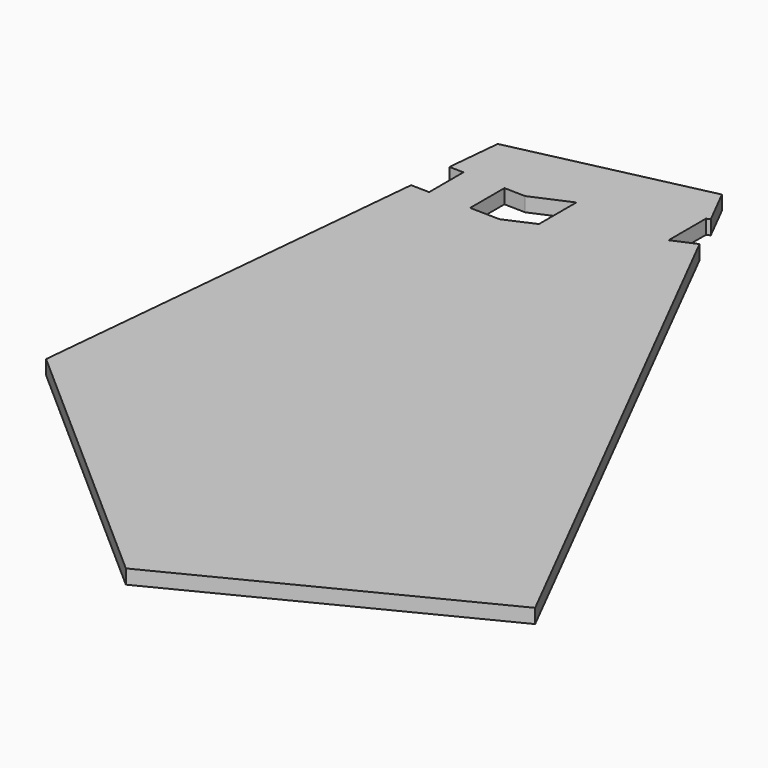
from build123d import *

# Parameters (mm, degrees)
F1_DEPTH = 1


# Not quite as in the source:
# - ends of sketch curves that miss each other by under 0.0002 mm in the source are joined


with BuildPart() as f1:
    # F0 (on Top) → F1 (new body)
    with BuildSketch(Plane.XY):
        Polygon((-2.198051, 23.051648), (-15.497051, 20.076648), (-15.856751674, 16.3066919689), (-14.8610655684, 16.2861461385), (-14.8610655684, 13.2855074428), (-16.1424234512, 13.311948043), (-18.862051, -15.198352), (0.006949, -31.811352), (20.3729486667, -21.4913521689), (0.507429, 17.711787), (-1.0988393333, 17.0108418244), (-1.0988393333, 20.2840446021), (-0.851051, 20.392648), align=None)
        Polygon((-11.9467116892, 16.2260088921), (-10.468051674, 16.1954969689), (-7.8843876222, 17.3229593784), (-7.8180441633, 17.3229593784), (-7.8180441633, 14.0787076895), (-9.871652, 13.182552), (-11.9467116892, 13.2253702503), align=None, mode=Mode.SUBTRACT)
    extrude(amount=F1_DEPTH)


solid = f1.part
